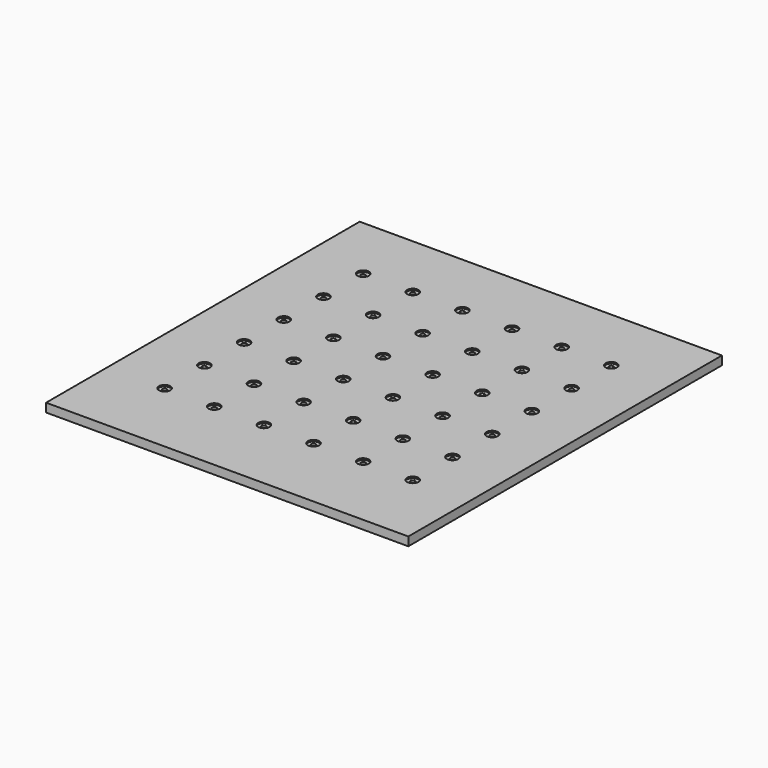
from build123d import *

# Parameters (mm, degrees)
F0_W           = 730
F0_H           = 790
F1_DEPTH       = 17.5
F3_D           = 9
F3_CBORE_D     = 23
F3_CBORE_DEPTH = 3


# Not quite as in the source:
# - a feature names something its author has since deleted; it is built from what else it names


with BuildPart() as f1:
    # F0 (on Top) → F1 (new body)
    with BuildSketch(Plane.XY):
        Rectangle(F0_W, F0_H)
    extrude(amount=F1_DEPTH)

    # F3 (through all)
    with Locations(Plane.XY.offset(17.5)):
        with Locations((-250, 260), (-150, 260), (-50, 260), (50, 260), (150, 260), (-150, 160), (-250, 60), (-250, 160), (150, 60), (-150, -140), (-150, -40), (150, -140), (50, -140), (-150, 60), (-50, 60), (-50, -140), (-250, -140), (50, 160), (50, -40), (-250, -40), (150, 160), (150, -40), (-50, 160), (-50, -40), (50, 60), (250, 260), (250, 160), (250, 60), (250, -40), (250, -140), (250, -240), (150, -240), (50, -240), (-50, -240), (-150, -240), (-250, -240)):
            CounterBoreHole(F3_D / 2, F3_CBORE_D / 2, F3_CBORE_DEPTH)


solid = f1.part
